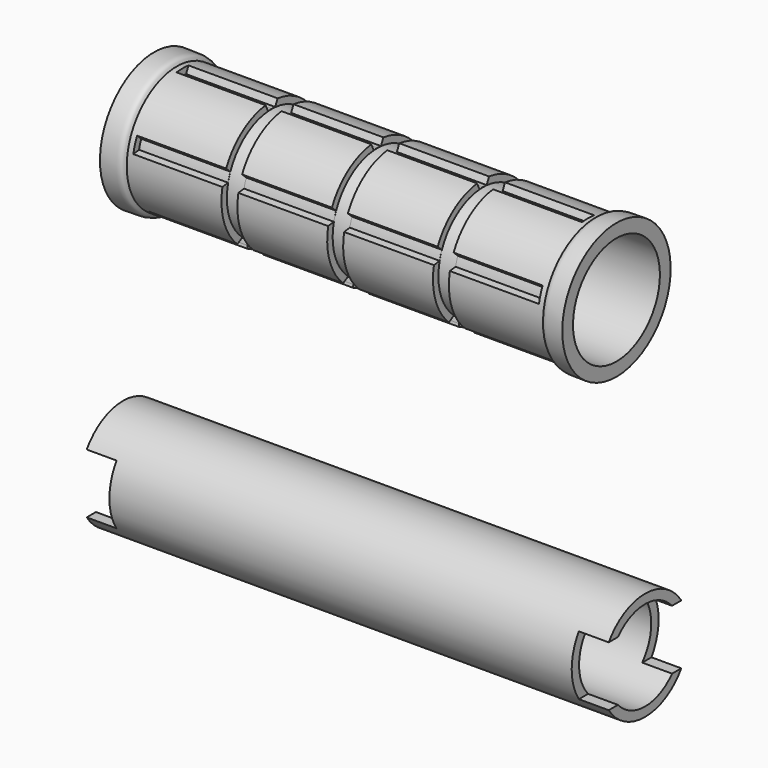
from build123d import *

# Parameters (mm, degrees)
F0_W     = 127.6
F0_H     = 2.25
F3_DEPTH = 15
F8_DEPTH = 49.57


with BuildPart() as f1:
    # F0 (on Front) → F1 (revolve)
    with BuildSketch(Plane.XZ):
        with Locations((63.8, 12.15)):
            Rectangle(F0_W, F0_H)
    revolve(axis=Axis((63.8, 0, 0), (1, 0, 0)))

    # F2 (on Front) → F3 (cut, symmetric)
    with BuildSketch(Plane.XZ):
        Polygon((120.3, 0.326546), (120.3, 0), (120.3, -7.3), (131.797016, -7.3), (131.797016, 0), (131.797016, 7.3), (120.3, 7.3), align=None)
        Polygon((7.3, -7.3), (7.3, 0), (7.3, 7.3), (-4.197016, 7.3), (-4.197016, 0), (-4.197016, -7.3), align=None)
    extrude(amount=F3_DEPTH, both=True, mode=Mode.SUBTRACT)


with BuildPart() as f5:
    # F4 (on Front) → F5 (revolve)
    with BuildSketch(Plane.XZ):
        with BuildLine():
            Line((120.617146, 60.949699), (7.617146, 60.949699))
            Line((7.617146, 60.949699), (7.617146, 58.909699))
            Line((7.617146, 58.909699), (7.617146, 57.664699))
            add(Edge.make_bspline(
                [(7.617146, 57.664699), (8.825806, 57.634047), (10.498774, 57.621826), (12.720447, 57.793691), (12.982954, 58.583933), (13.167146, 58.909699)],
                knots=[0, 0, 0, 0, 0.421301, 0.753212, 1, 1, 1, 1], degree=3))
            Line((13.167146, 58.909699), (36.317146, 58.909699))
            Line((36.317146, 58.909699), (36.317146, 60.574699))
            Line((36.317146, 60.574699), (40.217146, 60.574699))
            Line((40.217146, 60.574699), (40.217146, 58.909699))
            Line((40.217146, 58.909699), (62.167146, 58.909699))
            Line((62.167146, 58.909699), (62.167146, 60.574699))
            Line((62.167146, 60.574699), (66.067146, 60.574699))
            Line((66.067146, 60.574699), (66.067146, 58.909699))
            Line((66.067146, 58.909699), (88.017146, 58.909699))
            Line((88.017146, 58.909699), (88.017146, 60.574699))
            Line((88.017146, 60.574699), (91.917146, 60.574699))
            Line((91.917146, 60.574699), (91.917146, 58.909699))
            Line((91.917146, 58.909699), (115.067146, 58.909699))
            add(Edge.make_bspline(
                [(120.617146, 57.664699), (119.408487, 57.634047), (117.735519, 57.621826), (115.513846, 57.793691), (115.251339, 58.583933), (115.067146, 58.909699)],
                knots=[0, 0, 0, 0, 0.421301, 0.753212, 1, 1, 1, 1], degree=3))
            Line((120.617146, 57.664699), (120.617146, 58.909699))
            Line((120.617146, 58.909699), (120.617146, 60.949699))
        make_face()
    revolve(axis=Axis((64.117146, 0, 74.224699), (1, 0, 0)))

    # F7 (on offset) → F8 (cut, symmetric)
    with BuildSketch(Plane(origin=(64.117146, 0, 0), x_dir=(0, -1, 0), z_dir=(-1, 0, 0))):
        with BuildLine():
            ThreePointArc((0, 87.907433), (0.550448, 87.89633), (1.1, 87.863039))
            Line((1.1, 87.863039), (1.85, 89.460286))
            ThreePointArc((1.85, 89.460286), (0.926698, 89.544371), (0, 89.572433))
            ThreePointArc((0, 89.572433), (-0.926698, 89.544371), (-1.85, 89.460286))
            Line((-1.85, 89.460286), (-1.1, 87.863039))
            ThreePointArc((-1.1, 87.863039), (-0.550448, 87.89633), (0, 87.907433))
        make_face()
        with BuildLine():
            ThreePointArc((-13.279618, 77.415635), (-12.981921, 78.475515), (-12.599781, 79.507959))
            Line((-12.599781, 79.507959), (-13.887091, 80.714828))
            ThreePointArc((-13.887091, 80.714828), (-14.565431, 78.990029), (-15.030453, 77.195919))
            Line((-15.030453, 77.195919), (-13.279618, 77.415635))
        make_face()
        with BuildLine():
            ThreePointArc((-7.107256, 62.603704), (-8.023269, 63.214351), (-8.887093, 63.896831))
            Line((-8.887093, 63.896831), (-10.054141, 63.253988))
            Line((-10.054141, 63.253988), (-12.244109, 62.225671))
            Line((-12.244109, 62.225671), (-7.843184, 58.763035))
            Line((-7.843184, 58.763035), (-7.439331, 60.870665))
            Line((-7.439331, 60.870665), (-7.321163, 61.487363))
            Line((-7.321163, 61.487363), (-7.107256, 62.603704))
        make_face()
        with BuildLine():
            ThreePointArc((8.887093, 63.896831), (8.023269, 63.214351), (7.107256, 62.603704))
            Line((7.107256, 62.603704), (7.319633, 61.495344))
            Line((7.319633, 61.495344), (7.439331, 60.870665))
            Line((7.439331, 60.870665), (7.991223, 57.990447))
            Line((7.991223, 57.990447), (12.536565, 61.886598))
            Line((12.536565, 61.886598), (10.432694, 63.04547))
            Line((10.432694, 63.04547), (9.974365, 63.297931))
            Line((9.974365, 63.297931), (8.887093, 63.896831))
        make_face()
        with BuildLine():
            ThreePointArc((12.599781, 79.507959), (12.981921, 78.475515), (13.279618, 77.415635))
            Line((13.279618, 77.415635), (15.030453, 77.195919))
            ThreePointArc((15.030453, 77.195919), (14.565431, 78.990029), (13.887091, 80.714828))
            Line((13.887091, 80.714828), (12.599781, 79.507959))
        make_face()
    extrude(amount=F8_DEPTH, both=True, mode=Mode.SUBTRACT)


solid = Compound([f1.part, f5.part])
